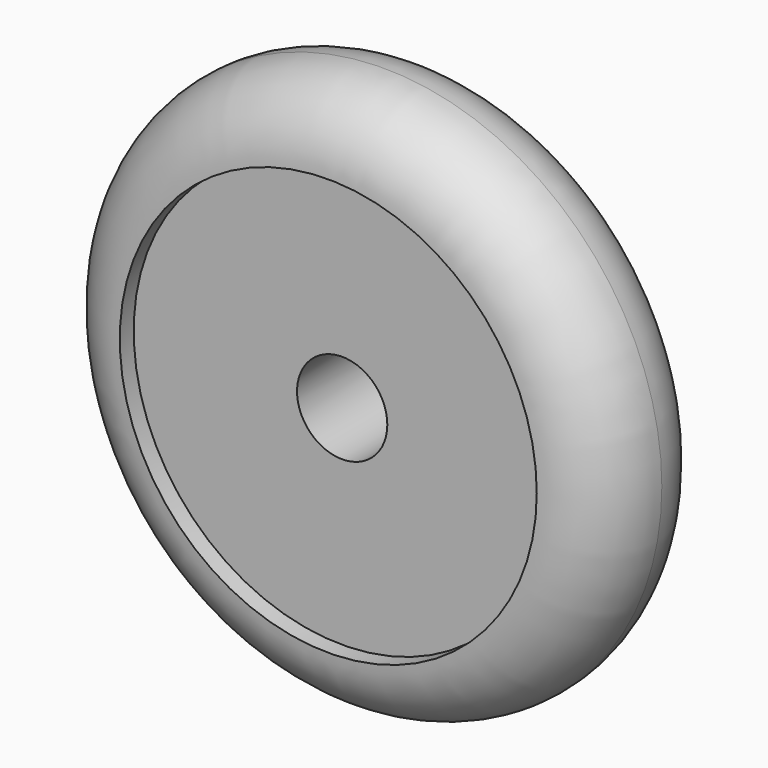
from build123d import *

# Parameters (mm, degrees)
F0_R     = 101.6
F1_DEPTH = 50.8
F2_R     = 25.39999
F3_R     = 16.5014152295
F4_DEPTH = 50.801
F5_DEPTH = 6.35
F6_DEPTH = 6.35


# Not quite as in the source:
# - a fillet or chamfer is up to 0.001 mm smaller than in the source, because OpenCascade refuses the exact size


with BuildPart() as f1:
    # F0 (on Front) → F1 (new body)
    with BuildSketch(Plane.XZ):
        Circle(F0_R)
    extrude(amount=F1_DEPTH)

    # F2 (radius 25.4 in the source; OpenCascade refuses exactly that, so slightly less here)
    f2_edges = [f1.edges().sort_by_distance(p)[0] for p in [
        (-101.6, -50.8, 0),
        (-101.6, 0, 0),
    ]]
    fillet(f2_edges, radius=F2_R)

    # F3 (on face) → F4 (cut, through all)
    with BuildSketch(Plane.XZ.offset(50.8)):
        Circle(F3_R)
    extrude(amount=-F4_DEPTH, mode=Mode.SUBTRACT)

    # F5 (cut): a face of the model
    f5_faces = [f1.faces().sort_by_distance(p)[0] for p in [
        (-74.0447482481, -50.8, 0),
    ]]
    extrude(f5_faces, amount=-F5_DEPTH, mode=Mode.SUBTRACT)

    # F6 (cut): a face of the model
    f6_faces = [f1.faces().sort_by_distance(p)[0] for p in [
        (-74.0447482481, 0, 0),
    ]]
    extrude(f6_faces, amount=-F6_DEPTH, mode=Mode.SUBTRACT)


solid = f1.part
